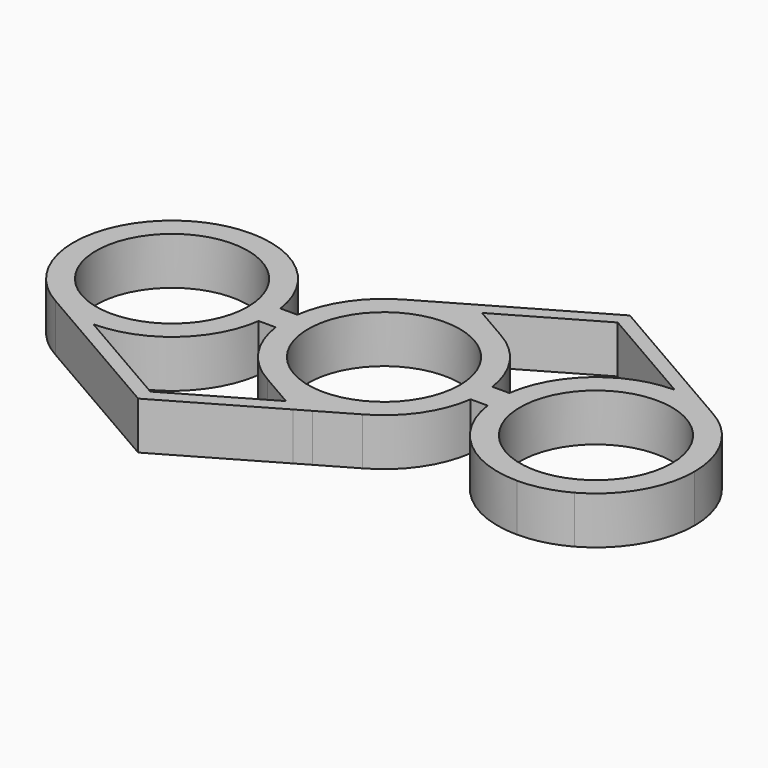
from build123d import *

# Parameters (mm, degrees)
F0_R     = 11.175
F1_DEPTH = 7


# Not quite as in the source:
# - a feature names something its author has since deleted; it is built from what else it names


with BuildPart() as f1:
    # F0 (on Top) → F1 (new body)
    with BuildSketch(Plane.XY):
        with BuildLine():
            ThreePointArc((14.3614066163, -2), (14.465310158, -1.0023981402), (14.5, 0))
            ThreePointArc((14.5, 0), (14.465310158, 1.0023981402), (14.3614066163, 2))
            ThreePointArc((14.3614066163, 2), (11.9468943762, 8.2171597748), (7.0047576617, 12.6958012784))
            ThreePointArc((7.0047576617, 12.6958012784), (3.6166891948, 14.0417078473), (0, 14.5))
            ThreePointArc((0, 14.5), (-3.6166891948, 14.0417078473), (-7.0047576617, 12.6958012784))
            ThreePointArc((-7.0047576617, 12.6958012784), (-11.9468943762, 8.2171597748), (-14.3614066163, 2))
            ThreePointArc((-14.3614066163, 2), (-14.5, 0), (-14.3614066163, -2))
            ThreePointArc((-14.3614066163, -2), (-11.9468943762, -8.2171597748), (-7.0047576617, -12.6958012784))
            ThreePointArc((-7.0047576617, -12.6958012784), (-3.6166891948, -14.0417078473), (0, -14.5))
            ThreePointArc((0, -14.5), (3.6166891948, -14.0417078473), (7.0047576617, -12.6958012784))
            ThreePointArc((7.0047576617, -12.6958012784), (11.9468943762, -8.2171597748), (14.3614066163, -2))
        make_face()
        Circle(F0_R, mode=Mode.SUBTRACT)
        with BuildLine():
            ThreePointArc((14.3614066163, 2), (14.465310158, 1.0023981402), (14.5, 0))
            ThreePointArc((14.5, 0), (14.465310158, -1.0023981402), (14.3614066163, -2))
            Line((14.3614066163, -2), (16.8614066163, -2))
            ThreePointArc((16.8614066163, -2), (16.7228132327, 0), (16.8614066163, 2))
            Line((16.8614066163, 2), (14.3614066163, 2))
        make_face()
        with BuildLine():
            ThreePointArc((0, 14.5), (3.6166891948, 14.0417078473), (7.0047576617, 12.6958012784))
            Line((7.0047576617, 12.6958012784), (1.9398969045, 15.62))
            Line((1.9398969045, 15.62), (0, 14.5))
        make_face()
        with BuildLine():
            ThreePointArc((31.2228132327, 14.5), (21.7030968504, 10.9373214271), (16.8614066163, 2))
            ThreePointArc((16.8614066163, 2), (16.7228132327, 0), (16.8614066163, -2))
            ThreePointArc((16.8614066163, -2), (21.7030968504, -10.9373214271), (31.2228132327, -14.5))
            ThreePointArc((31.2228132327, -14.5), (34.8395024275, -14.0417078473), (38.2275708944, -12.6958012784))
            ThreePointArc((38.2275708944, -12.6958012784), (43.709185526, -7.3716013832), (45.7228132327, 0))
            ThreePointArc((45.7228132327, 0), (43.709185526, 7.3716013832), (38.2275708944, 12.6958012784))
            ThreePointArc((38.2275708944, 12.6958012784), (34.8395024275, 14.0417078473), (31.2228132327, 14.5))
        make_face()
        with Locations((31.2228132327, 0)):
            Circle(F0_R, mode=Mode.SUBTRACT)
        with BuildLine():
            Line((1.9398969045, -15.62), (7.0047576617, -12.6958012784))
            ThreePointArc((7.0047576617, -12.6958012784), (3.6166891948, -14.0417078473), (0, -14.5))
            Line((0, -14.5), (1.9398969045, -15.62))
        make_face()
        Polygon((-1.9398969045, 15.62), (0, 14.5), (1.9398969045, 15.62), (0, 16.74), align=None)
        with BuildLine():
            ThreePointArc((-7.0047576617, 12.6958012784), (-3.6166891948, 14.0417078473), (0, 14.5))
            Line((0, 14.5), (-1.9398969045, 15.62))
            Line((-1.9398969045, 15.62), (-7.0047576617, 12.6958012784))
        make_face()
        Polygon((0, 16.74), (1.9398969045, 15.62), (15.6114066163, 23.5132498124), (15.6114066163, 25.7532498124), align=None)
        with BuildLine():
            Line((15.6114066163, 23.5132498124), (31.2228132327, 14.5))
            ThreePointArc((31.2228132327, 14.5), (34.8395024275, 14.0417078473), (38.2275708944, 12.6958012784))
            Line((38.2275708944, 12.6958012784), (15.6114066163, 25.7532498124))
            Line((15.6114066163, 25.7532498124), (15.6114066163, 23.5132498124))
        make_face()
        with BuildLine():
            Line((-1.9398969045, -15.62), (0, -14.5))
            ThreePointArc((0, -14.5), (-3.6166891948, -14.0417078473), (-7.0047576617, -12.6958012784))
            Line((-7.0047576617, -12.6958012784), (-1.9398969045, -15.62))
        make_face()
        Polygon((1.9398969045, -15.62), (0, -14.5), (-1.9398969045, -15.62), (0, -16.74), align=None)
        Polygon((0, -16.74), (-1.9398969045, -15.62), (-15.6114066163, -23.5132498124), (-15.6114066163, -25.7532498124), align=None)
        with BuildLine():
            ThreePointArc((-14.3614066163, -2), (-14.5, 0), (-14.3614066163, 2))
            Line((-14.3614066163, 2), (-16.8614066163, 2))
            ThreePointArc((-16.8614066163, 2), (-16.7575030746, 1.0023981402), (-16.7228132327, 0))
            ThreePointArc((-16.7228132327, 0), (-16.7575030746, -1.0023981402), (-16.8614066163, -2))
            Line((-16.8614066163, -2), (-14.3614066163, -2))
        make_face()
        with BuildLine():
            Line((-15.6114066163, -25.7532498124), (-15.6114066163, -23.5132498124))
            Line((-15.6114066163, -23.5132498124), (-31.2228132327, -14.5))
            ThreePointArc((-31.2228132327, -14.5), (-34.8395024275, -14.0417078473), (-38.2275708944, -12.6958012784))
            Line((-38.2275708944, -12.6958012784), (-15.6114066163, -25.7532498124))
        make_face()
        with BuildLine():
            ThreePointArc((-16.7228132327, 0), (-16.7575030746, 1.0023981402), (-16.8614066163, 2))
            ThreePointArc((-16.8614066163, 2), (-21.7030968504, 10.9373214271), (-31.2228132327, 14.5))
            ThreePointArc((-31.2228132327, 14.5), (-34.8395024275, 14.0417078473), (-38.2275708944, 12.6958012784))
            ThreePointArc((-38.2275708944, 12.6958012784), (-45.7228132327, 0), (-38.2275708944, -12.6958012784))
            ThreePointArc((-38.2275708944, -12.6958012784), (-34.8395024275, -14.0417078473), (-31.2228132327, -14.5))
            ThreePointArc((-31.2228132327, -14.5), (-21.7030968504, -10.9373214271), (-16.8614066163, -2))
            ThreePointArc((-16.8614066163, -2), (-16.7575030746, -1.0023981402), (-16.7228132327, 0))
        make_face()
        with Locations((-31.2228132327, 0)):
            Circle(F0_R, mode=Mode.SUBTRACT)
    extrude(amount=F1_DEPTH)


solid = f1.part
